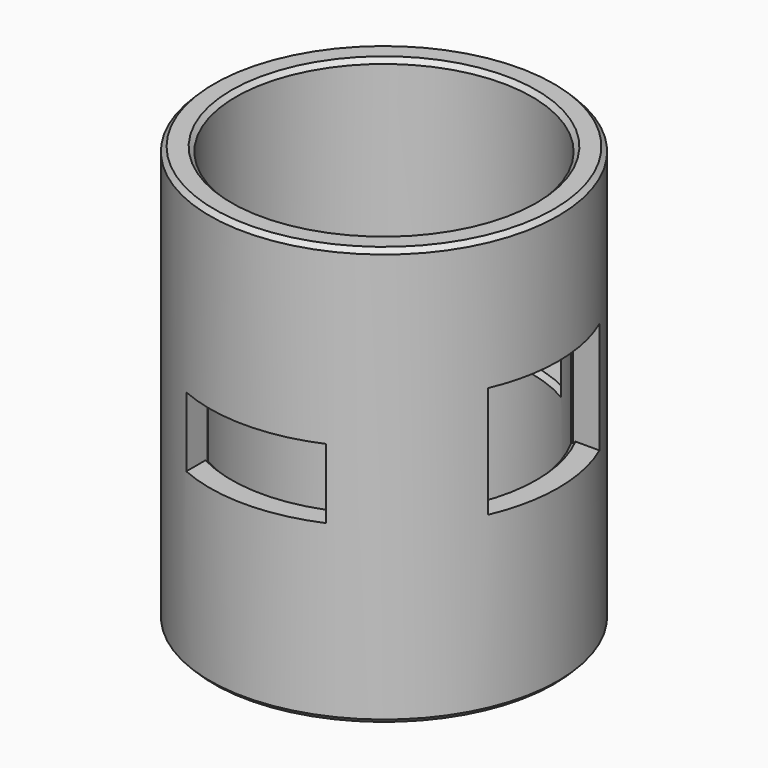
from build123d import *

# Parameters (mm, degrees)
F0_R          = 31.75
F0_R_2        = 26.9875
F1_DEPTH      = 76.2
F2_W          = 25.924757123
F2_H          = 12.7
F3_DEPTH      = 76.2
F4_W          = 25.4699392244
F4_H          = 12.7
F5_DEPTH      = 76.2
F6_W          = 25.4
F6_H          = 20.32
F7_DEPTH      = 76.2
F8_T1_DEPTH   = 20.32
F8_T3_DEPTH   = 12.7
F8_T8_ANGLE   = 32.5103926672
F8_T13_ANGLE  = 32.5103926672
F8_T18_ANGLE  = 32.5103926672
F8_T23_ANGLE  = 32.5103926672
F8_T28_ANGLE  = 66.292132353
F8_T34_ANGLE  = 66.292132353
F8_T40_ANGLE  = 65.190248715
F8_T46_ANGLE  = 65.190248715
F8_T53_ANGLE  = 32.5103926672
F8_T57_DEPTH  = 21.5976920802
F8_T64_ANGLE  = 32.5103926672
F8_T68_DEPTH  = 21.5976920802
F8_T75_ANGLE  = 32.5103926672
F8_T79_DEPTH  = 21.5976920802
F8_T86_DEPTH  = 21.5976920802
F8_T90_ANGLE  = 32.5103926672
F8_T97_ANGLE  = 66.292132353
F8_T101_DEPTH = 13.9481520643
F8_T108_ANGLE = 66.292132353
F8_T112_DEPTH = 13.9481520643
F8_T119_DEPTH = 13.9776920802
F8_T123_ANGLE = 66.292132353
F8_T130_DEPTH = 13.9776920802
F8_T134_ANGLE = 66.292132353
F8_T141_DEPTH = 13.9776920802
F8_T145_ANGLE = 65.190248715
F8_T152_DEPTH = 13.9776920802
F8_T156_ANGLE = 65.190248715
F8_T163_ANGLE = 65.190248715
F8_T167_DEPTH = 13.9737539479
F8_T174_ANGLE = 65.190248715
F8_T178_DEPTH = 13.9737539479
F9_SIZE       = 0.8128
F10_SIZE      = 1.6002


# Not quite as in the source:
# - a fillet or chamfer that OpenCascade refuses, or shapes differently, is made with other operations: its cross-section is extruded or revolved along the edge and cut away or added


with BuildPart() as f1:
    # F0 (on Top) → F1 (new body)
    with BuildSketch(Plane.XY):
        Circle(F0_R)
        Circle(F0_R_2, mode=Mode.SUBTRACT)
    extrude(amount=F1_DEPTH)

    # F2 (on Front) → F3 (cut)
    with BuildSketch(Plane.XZ):
        with Locations((0.2623785615, 38.1)):
            Rectangle(F2_W, F2_H)
    extrude(amount=-F3_DEPTH, mode=Mode.SUBTRACT)

    # F4 (on Front) → F5 (cut)
    with BuildSketch(Plane.XZ):
        with Locations((-0.0349696122, 38.1)):
            Rectangle(F4_W, F4_H)
    extrude(amount=F5_DEPTH, mode=Mode.SUBTRACT)

    # F6 (on Right) → F7 (cut)
    with BuildSketch(Plane.YZ):
        with Locations((0, 41.91)):
            Rectangle(F6_W, F6_H)
    extrude(amount=F7_DEPTH, mode=Mode.SUBTRACT)

    # F8: chamfer of 0.8128 on 14 edges, made by hand

    # F8_s2 → F8_t1 (cut)
    with BuildSketch(Plane.XY.offset(31.75)):
        with BuildLine():
            Line((24.2952858853, 12.7), (23.5849623144, 13.1177249886))
            ThreePointArc((23.5849623144, 13.1177249886), (23.6929781684, 12.9216075532), (23.8125, 12.7))
            Line((23.8125, 12.7), (24.2952858853, 12.7))
        make_face()
        with BuildLine():
            Line((24.2952858853, -12.7), (23.5849623144, -13.1177249886))
            ThreePointArc((23.5849623144, -13.1177249886), (23.6929781684, -12.9216075532), (23.8125, -12.7))
            Line((23.8125, -12.7), (24.2952858853, -12.7))
        make_face()
    extrude(amount=F8_T1_DEPTH, mode=Mode.SUBTRACT)

    # F8_s4 → F8_t3 (cut)
    with BuildSketch(Plane.XY.offset(31.75)):
        with BuildLine():
            Line((13.224757123, 23.9959094453), (13.6271397379, 23.2943387717))
            ThreePointArc((13.6271397379, 23.2943387717), (13.4386181576, 23.4036043862), (13.224757123, 23.5251132896))
            Line((13.224757123, 23.5251132896), (13.224757123, 23.9959094453))
        make_face()
        with BuildLine():
            Line((-12.7, 24.2952858853), (-13.1177249886, 23.5849623144))
            ThreePointArc((-13.1177249886, 23.5849623144), (-12.9216075532, 23.6929781684), (-12.7, 23.8125))
            Line((-12.7, 23.8125), (-12.7, 24.2952858853))
        make_face()
        with BuildLine():
            Line((12.7, -24.2952858853), (13.1177249886, -23.5849623144))
            ThreePointArc((13.1177249886, -23.5849623144), (12.9216075532, -23.6929781684), (12.7, -23.8125))
            Line((12.7, -23.8125), (12.7, -24.2952858853))
        make_face()
        with BuildLine():
            Line((-12.7699392244, -24.2562543533), (-13.1856193933, -23.547071951))
            ThreePointArc((-13.1856193933, -23.547071951), (-12.9905149919, -23.6552674154), (-12.7699392244, -23.7750669495))
            Line((-12.7699392244, -23.7750669495), (-12.7699392244, -24.2562543533))
        make_face()
    extrude(amount=F8_T3_DEPTH, mode=Mode.SUBTRACT)


with BuildPart() as f8_tool6:
    # F8_s7 → F8_t8 (revolve)
    with BuildSketch(Plane.XZ):
        Polygon((27.8003, 31.75), (26.9875, 30.9372), (26.9875, 31.75), align=None)
    revolve(axis=Axis((0, 0, 31.75), (0, 0, -1)), revolution_arc=F8_T8_ANGLE)

    split(bisect_by=Plane.XZ.offset(12.7), keep=Keep.BOTTOM)


with BuildPart() as f1_1:
    add(f1.part)

    # F8_t5: cut F8_tool6
    add(f8_tool6.part, mode=Mode.SUBTRACT)


with BuildPart() as f8_tool11:
    # F8_s12 → F8_t13 (revolve)
    with BuildSketch(Plane(origin=(0, 0, 0), x_dir=(0, 0, 1), z_dir=(-0.5374525791, 0.8432939732, 0))):
        Polygon((31.75, 27.8003), (30.9372, 26.9875), (31.75, 26.9875), align=None)
    revolve(axis=Axis((0, 0, 31.75), (0, 0, -1)), revolution_arc=F8_T13_ANGLE)

    split(bisect_by=Plane.XZ.offset(-12.7), keep=Keep.TOP)


with BuildPart() as f1_2:
    add(f1_1.part)

    # F8_t10: cut F8_tool11
    add(f8_tool11.part, mode=Mode.SUBTRACT)


with BuildPart() as f8_tool16:
    # F8_s17 → F8_t18 (revolve)
    with BuildSketch(Plane.XZ):
        Polygon((27.8003, 52.07), (26.9875, 52.8828), (26.9875, 52.07), align=None)
    revolve(axis=Axis((0, 0, 52.07), (0, 0, -1)), revolution_arc=F8_T18_ANGLE)

    split(bisect_by=Plane.XZ.offset(12.7), keep=Keep.BOTTOM)


with BuildPart() as f1_3:
    add(f1_2.part)

    # F8_t15: cut F8_tool16
    add(f8_tool16.part, mode=Mode.SUBTRACT)


with BuildPart() as f8_tool21:
    # F8_s22 → F8_t23 (revolve)
    with BuildSketch(Plane(origin=(0, 0, 0), x_dir=(0, 0, 1), z_dir=(-0.5374525791, 0.8432939732, 0))):
        Polygon((52.07, 27.8003), (52.8828, 26.9875), (52.07, 26.9875), align=None)
    revolve(axis=Axis((0, 0, 52.07), (0, 0, -1)), revolution_arc=F8_T23_ANGLE)

    split(bisect_by=Plane.XZ.offset(-12.7), keep=Keep.TOP)


with BuildPart() as f1_4:
    add(f1_3.part)

    # F8_t20: cut F8_tool21
    add(f8_tool21.part, mode=Mode.SUBTRACT)


with BuildPart() as f8_tool26:
    # F8_s27 → F8_t28 (revolve)
    with BuildSketch(Plane(origin=(0, 0, 0), x_dir=(0, 0, 1), z_dir=(-0.8432887953, -0.5374607034, 0))):
        Polygon((31.75, 27.8003), (30.9372, 26.9875), (31.75, 26.9875), align=None)
    revolve(axis=Axis((0, 0, 31.75), (0, 0, -1)), revolution_arc=F8_T28_ANGLE)

    split(bisect_by=Plane.YZ.offset(-12.7), keep=Keep.TOP)

    split(bisect_by=Plane.YZ.offset(13.224757123), keep=Keep.BOTTOM)


with BuildPart() as f1_5:
    add(f1_4.part)

    # F8_t25: cut F8_tool26
    add(f8_tool26.part, mode=Mode.SUBTRACT)


with BuildPart() as f8_tool32:
    # F8_s33 → F8_t34 (revolve)
    with BuildSketch(Plane(origin=(0, 0, 0), x_dir=(0, 0, 1), z_dir=(-0.8432887953, -0.5374607034, 0))):
        Polygon((44.45, 27.8003), (45.2628, 26.9875), (44.45, 26.9875), align=None)
    revolve(axis=Axis((0, 0, 44.45), (0, 0, -1)), revolution_arc=F8_T34_ANGLE)

    split(bisect_by=Plane.YZ.offset(-12.7), keep=Keep.TOP)

    split(bisect_by=Plane.YZ.offset(13.224757123), keep=Keep.BOTTOM)


with BuildPart() as f1_6:
    add(f1_5.part)

    # F8_t31: cut F8_tool32
    add(f8_tool32.part, mode=Mode.SUBTRACT)


with BuildPart() as f8_tool38:
    # F8_s39 → F8_t40 (revolve)
    with BuildSketch(Plane(origin=(0, 0, 0), x_dir=(0, 0, 1), z_dir=(0.843289054, 0.5374602975, 0))):
        Polygon((31.75, 27.8003), (30.9372, 26.9875), (31.75, 26.9875), align=None)
    revolve(axis=Axis((0, 0, 31.75), (0, 0, -1)), revolution_arc=F8_T40_ANGLE)

    split(bisect_by=Plane.YZ.offset(12.7), keep=Keep.BOTTOM)

    split(bisect_by=Plane.YZ.offset(-12.7699392244), keep=Keep.TOP)


with BuildPart() as f1_7:
    add(f1_6.part)

    # F8_t37: cut F8_tool38
    add(f8_tool38.part, mode=Mode.SUBTRACT)


with BuildPart() as f8_tool44:
    # F8_s45 → F8_t46 (revolve)
    with BuildSketch(Plane(origin=(0, 0, 0), x_dir=(0, 0, 1), z_dir=(0.843289054, 0.5374602975, 0))):
        Polygon((44.45, 27.8003), (45.2628, 26.9875), (44.45, 26.9875), align=None)
    revolve(axis=Axis((0, 0, 44.45), (0, 0, -1)), revolution_arc=F8_T46_ANGLE)

    split(bisect_by=Plane.YZ.offset(12.7), keep=Keep.BOTTOM)

    split(bisect_by=Plane.YZ.offset(-12.7699392244), keep=Keep.TOP)


with BuildPart() as f1_8:
    add(f1_7.part)

    # F8_t43: cut F8_tool44
    add(f8_tool44.part, mode=Mode.SUBTRACT)


with BuildPart() as f8_tool51:
    # F8_s52 → F8_t53 (revolve)
    with BuildSketch(Plane.XZ):
        Polygon((27.8003, 31.75), (26.9875, 30.9372), (26.9875, 31.75), align=None)
    revolve(axis=Axis((0, 0, 31.75), (0, 0, -1)), revolution_arc=F8_T53_ANGLE)

    split(bisect_by=Plane.XZ.offset(12.7), keep=Keep.TOP)


with BuildPart() as f8_tool55:
    # F8_s56 → F8_t57 (new body)
    with BuildSketch(Plane.XY.offset(52.07)):
        with BuildLine():
            Line((24.2952858853, -12.7), (23.5849623144, -13.1177249886))
            ThreePointArc((23.5849623144, -13.1177249886), (23.6929781684, -12.9216075532), (23.8125, -12.7))
            Line((23.8125, -12.7), (24.2952858853, -12.7))
        make_face()
    extrude(amount=-F8_T57_DEPTH)

    split(bisect_by=Plane.XY.offset(31.75), keep=Keep.BOTTOM)


with BuildPart() as f8_tool51_1:
    add(f8_tool51.part)

    # F8_t59: intersect F8_tool55
    add(f8_tool55.part, mode=Mode.INTERSECT)


with BuildPart() as f1_9:
    add(f1_8.part)

    # F8_t49: cut F8_tool51
    add(f8_tool51_1.part, mode=Mode.SUBTRACT)


with BuildPart() as f8_tool62:
    # F8_s63 → F8_t64 (revolve)
    with BuildSketch(Plane(origin=(0, 0, 0), x_dir=(0, 0, 1), z_dir=(-0.5374525791, 0.8432939732, 0))):
        Polygon((31.75, 27.8003), (30.9372, 26.9875), (31.75, 26.9875), align=None)
    revolve(axis=Axis((0, 0, 31.75), (0, 0, -1)), revolution_arc=F8_T64_ANGLE)

    split(bisect_by=Plane.XZ.offset(-12.7), keep=Keep.BOTTOM)


with BuildPart() as f8_tool66:
    # F8_s67 → F8_t68 (new body)
    with BuildSketch(Plane.XY.offset(52.07)):
        with BuildLine():
            Line((24.2952858853, 12.7), (23.5849623144, 13.1177249886))
            ThreePointArc((23.5849623144, 13.1177249886), (23.6929781684, 12.9216075532), (23.8125, 12.7))
            Line((23.8125, 12.7), (24.2952858853, 12.7))
        make_face()
    extrude(amount=-F8_T68_DEPTH)

    split(bisect_by=Plane.XY.offset(31.75), keep=Keep.BOTTOM)


with BuildPart() as f8_tool62_1:
    add(f8_tool62.part)

    # F8_t70: intersect F8_tool66
    add(f8_tool66.part, mode=Mode.INTERSECT)


with BuildPart() as f1_10:
    add(f1_9.part)

    # F8_t60: cut F8_tool62
    add(f8_tool62_1.part, mode=Mode.SUBTRACT)


with BuildPart() as f8_tool73:
    # F8_s74 → F8_t75 (revolve)
    with BuildSketch(Plane(origin=(0, 0, 0), x_dir=(0, 0, 1), z_dir=(-0.5374525791, 0.8432939732, 0))):
        Polygon((52.07, 27.8003), (52.8828, 26.9875), (52.07, 26.9875), align=None)
    revolve(axis=Axis((0, 0, 52.07), (0, 0, -1)), revolution_arc=F8_T75_ANGLE)

    split(bisect_by=Plane.XZ.offset(-12.7), keep=Keep.BOTTOM)


with BuildPart() as f8_tool77:
    # F8_s78 → F8_t79 (new body)
    with BuildSketch(Plane.XY.offset(53.3476920802)):
        with BuildLine():
            Line((24.2952858853, 12.7), (23.5849623144, 13.1177249886))
            ThreePointArc((23.5849623144, 13.1177249886), (23.6929781684, 12.9216075532), (23.8125, 12.7))
            Line((23.8125, 12.7), (24.2952858853, 12.7))
        make_face()
    extrude(amount=-F8_T79_DEPTH)

    split(bisect_by=Plane.XY.offset(52.07), keep=Keep.TOP)


with BuildPart() as f8_tool73_1:
    add(f8_tool73.part)

    # F8_t81: intersect F8_tool77
    add(f8_tool77.part, mode=Mode.INTERSECT)


with BuildPart() as f1_11:
    add(f1_10.part)

    # F8_t71: cut F8_tool73
    add(f8_tool73_1.part, mode=Mode.SUBTRACT)


with BuildPart() as f8_tool84:
    # F8_s85 → F8_t86 (new body)
    with BuildSketch(Plane.XY.offset(53.3476920802)):
        with BuildLine():
            Line((24.2952858853, -12.7), (23.5849623144, -13.1177249886))
            ThreePointArc((23.5849623144, -13.1177249886), (23.6929781684, -12.9216075532), (23.8125, -12.7))
            Line((23.8125, -12.7), (24.2952858853, -12.7))
        make_face()
    extrude(amount=-F8_T86_DEPTH)

    split(bisect_by=Plane.XY.offset(52.07), keep=Keep.TOP)


with BuildPart() as f8_tool88:
    # F8_s89 → F8_t90 (revolve)
    with BuildSketch(Plane.XZ):
        Polygon((27.8003, 52.07), (26.9875, 52.8828), (26.9875, 52.07), align=None)
    revolve(axis=Axis((0, 0, 52.07), (0, 0, -1)), revolution_arc=F8_T90_ANGLE)

    split(bisect_by=Plane.XZ.offset(12.7), keep=Keep.TOP)


with BuildPart() as f8_tool84_1:
    add(f8_tool84.part)

    # F8_t92: intersect F8_tool88
    add(f8_tool88.part, mode=Mode.INTERSECT)


with BuildPart() as f1_12:
    add(f1_11.part)

    # F8_t82: cut F8_tool84
    add(f8_tool84_1.part, mode=Mode.SUBTRACT)


with BuildPart() as f8_tool95:
    # F8_s96 → F8_t97 (revolve)
    with BuildSketch(Plane(origin=(0, 0, 0), x_dir=(0, 0, 1), z_dir=(-0.8432887953, -0.5374607034, 0))):
        Polygon((44.45, 27.8003), (45.2628, 26.9875), (44.45, 26.9875), align=None)
    revolve(axis=Axis((0, 0, 44.45), (0, 0, -1)), revolution_arc=F8_T97_ANGLE)

    split(bisect_by=Plane.YZ.offset(13.224757123), keep=Keep.TOP)


with BuildPart() as f8_tool99:
    # F8_s100 → F8_t101 (new body)
    with BuildSketch(Plane.XY.offset(45.6981520643)):
        with BuildLine():
            Line((13.224757123, 23.9959094453), (13.6271397379, 23.2943387717))
            ThreePointArc((13.6271397379, 23.2943387717), (13.4386181576, 23.4036043862), (13.224757123, 23.5251132896))
            Line((13.224757123, 23.5251132896), (13.224757123, 23.9959094453))
        make_face()
    extrude(amount=-F8_T101_DEPTH)

    split(bisect_by=Plane.XY.offset(44.45), keep=Keep.TOP)


with BuildPart() as f8_tool95_1:
    add(f8_tool95.part)

    # F8_t103: intersect F8_tool99
    add(f8_tool99.part, mode=Mode.INTERSECT)


with BuildPart() as f1_13:
    add(f1_12.part)

    # F8_t93: cut F8_tool95
    add(f8_tool95_1.part, mode=Mode.SUBTRACT)


with BuildPart() as f8_tool106:
    # F8_s107 → F8_t108 (revolve)
    with BuildSketch(Plane(origin=(0, 0, 0), x_dir=(0, 0, 1), z_dir=(-0.8432887953, -0.5374607034, 0))):
        Polygon((31.75, 27.8003), (30.9372, 26.9875), (31.75, 26.9875), align=None)
    revolve(axis=Axis((0, 0, 31.75), (0, 0, -1)), revolution_arc=F8_T108_ANGLE)

    split(bisect_by=Plane.YZ.offset(13.224757123), keep=Keep.TOP)


with BuildPart() as f8_tool110:
    # F8_s111 → F8_t112 (new body)
    with BuildSketch(Plane.XY.offset(44.45)):
        with BuildLine():
            Line((13.224757123, 23.9959094453), (13.6271397379, 23.2943387717))
            ThreePointArc((13.6271397379, 23.2943387717), (13.4386181576, 23.4036043862), (13.224757123, 23.5251132896))
            Line((13.224757123, 23.5251132896), (13.224757123, 23.9959094453))
        make_face()
    extrude(amount=-F8_T112_DEPTH)

    split(bisect_by=Plane.XY.offset(31.75), keep=Keep.BOTTOM)


with BuildPart() as f8_tool106_1:
    add(f8_tool106.part)

    # F8_t114: intersect F8_tool110
    add(f8_tool110.part, mode=Mode.INTERSECT)


with BuildPart() as f1_14:
    add(f1_13.part)

    # F8_t104: cut F8_tool106
    add(f8_tool106_1.part, mode=Mode.SUBTRACT)


with BuildPart() as f8_tool117:
    # F8_s118 → F8_t119 (new body)
    with BuildSketch(Plane.XY.offset(44.45)):
        with BuildLine():
            Line((-12.7, 24.2952858853), (-13.1177249886, 23.5849623144))
            ThreePointArc((-13.1177249886, 23.5849623144), (-12.9216075532, 23.6929781684), (-12.7, 23.8125))
            Line((-12.7, 23.8125), (-12.7, 24.2952858853))
        make_face()
    extrude(amount=-F8_T119_DEPTH)

    split(bisect_by=Plane.XY.offset(31.75), keep=Keep.BOTTOM)


with BuildPart() as f8_tool121:
    # F8_s122 → F8_t123 (revolve)
    with BuildSketch(Plane(origin=(0, 0, 0), x_dir=(0, 0, 1), z_dir=(-0.8432887953, -0.5374607034, 0))):
        Polygon((31.75, 27.8003), (30.9372, 26.9875), (31.75, 26.9875), align=None)
    revolve(axis=Axis((0, 0, 31.75), (0, 0, -1)), revolution_arc=F8_T123_ANGLE)

    split(bisect_by=Plane.YZ.offset(-12.7), keep=Keep.BOTTOM)


with BuildPart() as f8_tool117_1:
    add(f8_tool117.part)

    # F8_t125: intersect F8_tool121
    add(f8_tool121.part, mode=Mode.INTERSECT)


with BuildPart() as f1_15:
    add(f1_14.part)

    # F8_t115: cut F8_tool117
    add(f8_tool117_1.part, mode=Mode.SUBTRACT)


with BuildPart() as f8_tool128:
    # F8_s129 → F8_t130 (new body)
    with BuildSketch(Plane.XY.offset(45.7276920802)):
        with BuildLine():
            Line((-12.7, 24.2952858853), (-13.1177249886, 23.5849623144))
            ThreePointArc((-13.1177249886, 23.5849623144), (-12.9216075532, 23.6929781684), (-12.7, 23.8125))
            Line((-12.7, 23.8125), (-12.7, 24.2952858853))
        make_face()
    extrude(amount=-F8_T130_DEPTH)

    split(bisect_by=Plane.XY.offset(44.45), keep=Keep.TOP)


with BuildPart() as f8_tool132:
    # F8_s133 → F8_t134 (revolve)
    with BuildSketch(Plane(origin=(0, 0, 0), x_dir=(0, 0, 1), z_dir=(-0.8432887953, -0.5374607034, 0))):
        Polygon((44.45, 27.8003), (45.2628, 26.9875), (44.45, 26.9875), align=None)
    revolve(axis=Axis((0, 0, 44.45), (0, 0, -1)), revolution_arc=F8_T134_ANGLE)

    split(bisect_by=Plane.YZ.offset(-12.7), keep=Keep.BOTTOM)


with BuildPart() as f8_tool128_1:
    add(f8_tool128.part)

    # F8_t136: intersect F8_tool132
    add(f8_tool132.part, mode=Mode.INTERSECT)


with BuildPart() as f1_16:
    add(f1_15.part)

    # F8_t126: cut F8_tool128
    add(f8_tool128_1.part, mode=Mode.SUBTRACT)


with BuildPart() as f8_tool139:
    # F8_s140 → F8_t141 (new body)
    with BuildSketch(Plane.XY.offset(45.7276920802)):
        with BuildLine():
            Line((12.7, -24.2952858853), (13.1177249886, -23.5849623144))
            ThreePointArc((13.1177249886, -23.5849623144), (12.9216075532, -23.6929781684), (12.7, -23.8125))
            Line((12.7, -23.8125), (12.7, -24.2952858853))
        make_face()
    extrude(amount=-F8_T141_DEPTH)

    split(bisect_by=Plane.XY.offset(44.45), keep=Keep.TOP)


with BuildPart() as f8_tool143:
    # F8_s144 → F8_t145 (revolve)
    with BuildSketch(Plane(origin=(0, 0, 0), x_dir=(0, 0, 1), z_dir=(0.843289054, 0.5374602975, 0))):
        Polygon((44.45, 27.8003), (45.2628, 26.9875), (44.45, 26.9875), align=None)
    revolve(axis=Axis((0, 0, 44.45), (0, 0, -1)), revolution_arc=F8_T145_ANGLE)

    split(bisect_by=Plane.YZ.offset(12.7), keep=Keep.TOP)


with BuildPart() as f8_tool139_1:
    add(f8_tool139.part)

    # F8_t147: intersect F8_tool143
    add(f8_tool143.part, mode=Mode.INTERSECT)


with BuildPart() as f1_17:
    add(f1_16.part)

    # F8_t137: cut F8_tool139
    add(f8_tool139_1.part, mode=Mode.SUBTRACT)


with BuildPart() as f8_tool150:
    # F8_s151 → F8_t152 (new body)
    with BuildSketch(Plane.XY.offset(44.45)):
        with BuildLine():
            Line((12.7, -24.2952858853), (13.1177249886, -23.5849623144))
            ThreePointArc((13.1177249886, -23.5849623144), (12.9216075532, -23.6929781684), (12.7, -23.8125))
            Line((12.7, -23.8125), (12.7, -24.2952858853))
        make_face()
    extrude(amount=-F8_T152_DEPTH)

    split(bisect_by=Plane.XY.offset(31.75), keep=Keep.BOTTOM)


with BuildPart() as f8_tool154:
    # F8_s155 → F8_t156 (revolve)
    with BuildSketch(Plane(origin=(0, 0, 0), x_dir=(0, 0, 1), z_dir=(0.843289054, 0.5374602975, 0))):
        Polygon((31.75, 27.8003), (30.9372, 26.9875), (31.75, 26.9875), align=None)
    revolve(axis=Axis((0, 0, 31.75), (0, 0, -1)), revolution_arc=F8_T156_ANGLE)

    split(bisect_by=Plane.YZ.offset(12.7), keep=Keep.TOP)


with BuildPart() as f8_tool150_1:
    add(f8_tool150.part)

    # F8_t158: intersect F8_tool154
    add(f8_tool154.part, mode=Mode.INTERSECT)


with BuildPart() as f1_18:
    add(f1_17.part)

    # F8_t148: cut F8_tool150
    add(f8_tool150_1.part, mode=Mode.SUBTRACT)


with BuildPart() as f8_tool161:
    # F8_s162 → F8_t163 (revolve)
    with BuildSketch(Plane(origin=(0, 0, 0), x_dir=(0, 0, 1), z_dir=(0.843289054, 0.5374602975, 0))):
        Polygon((44.45, 27.8003), (45.2628, 26.9875), (44.45, 26.9875), align=None)
    revolve(axis=Axis((0, 0, 44.45), (0, 0, -1)), revolution_arc=F8_T163_ANGLE)

    split(bisect_by=Plane.YZ.offset(-12.7699392244), keep=Keep.BOTTOM)


with BuildPart() as f8_tool165:
    # F8_s166 → F8_t167 (new body)
    with BuildSketch(Plane.XY.offset(45.7237539479)):
        with BuildLine():
            Line((-12.7699392244, -24.2562543533), (-13.1856193933, -23.547071951))
            ThreePointArc((-13.1856193933, -23.547071951), (-12.9905149919, -23.6552674154), (-12.7699392244, -23.7750669495))
            Line((-12.7699392244, -23.7750669495), (-12.7699392244, -24.2562543533))
        make_face()
    extrude(amount=-F8_T167_DEPTH)

    split(bisect_by=Plane.XY.offset(44.45), keep=Keep.TOP)


with BuildPart() as f8_tool161_1:
    add(f8_tool161.part)

    # F8_t169: intersect F8_tool165
    add(f8_tool165.part, mode=Mode.INTERSECT)


with BuildPart() as f1_19:
    add(f1_18.part)

    # F8_t159: cut F8_tool161
    add(f8_tool161_1.part, mode=Mode.SUBTRACT)


with BuildPart() as f8_tool172:
    # F8_s173 → F8_t174 (revolve)
    with BuildSketch(Plane(origin=(0, 0, 0), x_dir=(0, 0, 1), z_dir=(0.843289054, 0.5374602975, 0))):
        Polygon((31.75, 27.8003), (30.9372, 26.9875), (31.75, 26.9875), align=None)
    revolve(axis=Axis((0, 0, 31.75), (0, 0, -1)), revolution_arc=F8_T174_ANGLE)

    split(bisect_by=Plane.YZ.offset(-12.7699392244), keep=Keep.BOTTOM)


with BuildPart() as f8_tool176:
    # F8_s177 → F8_t178 (new body)
    with BuildSketch(Plane.XY.offset(44.45)):
        with BuildLine():
            Line((-12.7699392244, -24.2562543533), (-13.1856193933, -23.547071951))
            ThreePointArc((-13.1856193933, -23.547071951), (-12.9905149919, -23.6552674154), (-12.7699392244, -23.7750669495))
            Line((-12.7699392244, -23.7750669495), (-12.7699392244, -24.2562543533))
        make_face()
    extrude(amount=-F8_T178_DEPTH)

    split(bisect_by=Plane.XY.offset(31.75), keep=Keep.BOTTOM)


with BuildPart() as f8_tool172_1:
    add(f8_tool172.part)

    # F8_t180: intersect F8_tool176
    add(f8_tool176.part, mode=Mode.INTERSECT)


with BuildPart() as f1_20:
    add(f1_19.part)

    # F8_t170: cut F8_tool172
    add(f8_tool172_1.part, mode=Mode.SUBTRACT)

    # F9
    f9_edges = [f1_20.edges().sort_by_distance(p)[0] for p in [
        (-26.9875, 0, 76.2),
        (-31.75, 0, 76.2),
        (-31.75, 0, 0),
    ]]
    chamfer(f9_edges, length=F9_SIZE)

    # F10
    f10_edges = [f1_20.edges().sort_by_distance(p)[0] for p in [
        (-26.9875, 0, 0),
    ]]
    chamfer(f10_edges, length=F10_SIZE)


solid = f1_20.part
